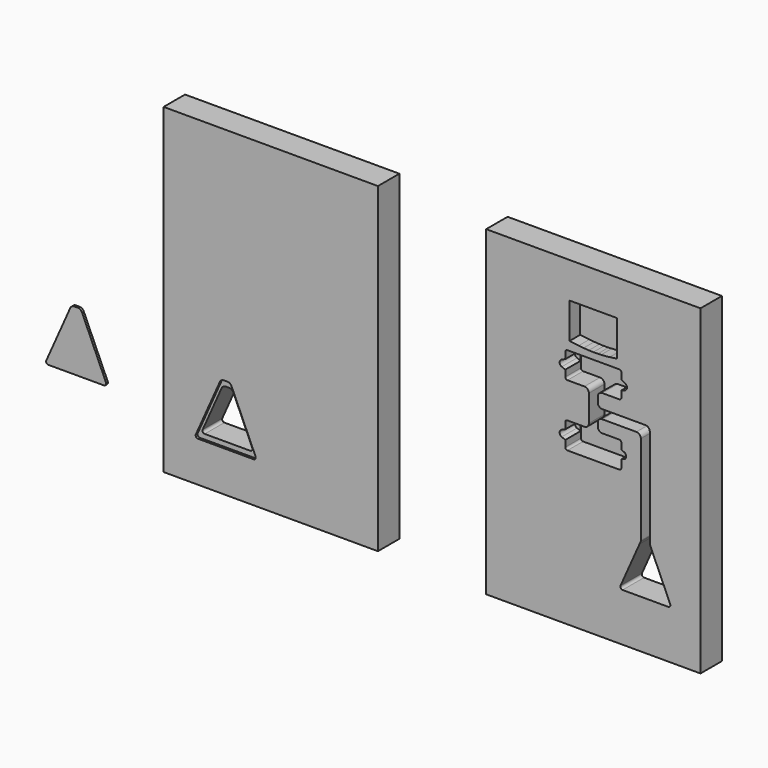
from build123d import *

# Parameters (mm, degrees)
F1_DEPTH = 38.1
F0_W     = 304.8
F0_H     = 457.2
F2_DEPTH = 10.383012
F3_DEPTH = 10.891012
F4_DEPTH = 19.05
F5_DEPTH = 34.925
F6_DEPTH = 3.175


# Not quite as in the source:
# - a feature names something its author has since deleted; it is built from what else it names


with BuildPart() as f1:
    # F0 (on Front) → F1 (new body)
    with BuildSketch(Plane.XZ):
        Polygon((-152.3615987246, 208.8922339559), (-152.3615987246, -197.5077660441), (152.4384012754, -197.5077660441), (152.4384012754, 208.8922339559), (152.4384012754, 259.6922339559), (-152.3615987246, 259.6922339559), align=None)
        with BuildLine():
            ThreePointArc((-39.8395987246, 54.7480871081), (-38.9468601937, 56.9033485772), (-36.7915987246, 57.7960871081))
            Line((-36.7915987246, 57.7960871081), (-12.6615987246, 57.7960871081))
            ThreePointArc((-12.6615987246, 57.7960871081), (-8.1714706641, 59.6559590476), (-6.3115987246, 64.1460871081))
            Line((-6.3115987246, 64.1460871081), (-6.3115987246, 101.8113421874))
            ThreePointArc((-6.3115987246, 101.8113421874), (-8.1714706641, 106.3014702479), (-12.6615987246, 108.1613421874))
            Line((-12.6615987246, 108.1613421874), (-36.7915987246, 108.1613421874))
            ThreePointArc((-36.7915987246, 108.1613421874), (-38.9468601937, 109.0540807183), (-39.8395987246, 111.2093421874))
            Line((-39.8395987246, 111.2093421874), (-39.8395987246, 120.3533421874))
            Line((-39.8395987246, 120.3533421874), (-44.9068001558, 122.3898638359))
            ThreePointArc((-44.9068001558, 122.3898638359), (-47.9325949829, 126.7961256548), (-45.0389055671, 131.2902483852))
            Line((-45.0389055671, 131.2902483852), (-39.8395987246, 133.5613421874))
            Line((-39.8395987246, 133.5613421874), (-39.8395987246, 142.7053421874))
            ThreePointArc((-39.8395987246, 142.7053421874), (-38.9468601937, 144.8606036565), (-36.7915987246, 145.7533421874))
            Line((-36.7915987246, 145.7533421874), (36.8684012754, 145.7533421874))
            ThreePointArc((36.8684012754, 145.7533421874), (39.0236627444, 144.8606036565), (39.9164012754, 142.7053421874))
            Line((39.9164012754, 142.7053421874), (39.9164012754, 133.5613421874))
            Line((39.9164012754, 133.5613421874), (45.3107705248, 130.8709577364))
            ThreePointArc((45.3107705248, 130.8709577364), (47.971895997, 126.2269453196), (44.7102550148, 121.9831100014))
            Line((44.7102550148, 121.9831100014), (39.9164012754, 120.3533421874))
            Line((39.9164012754, 120.3533421874), (39.9164012754, 111.2093421874))
            ThreePointArc((39.9164012754, 111.2093421874), (39.0236627444, 109.0540807183), (36.8684012754, 108.1613421874))
            Line((36.8684012754, 108.1613421874), (12.7384012754, 108.1613421874))
            ThreePointArc((12.7384012754, 108.1613421874), (8.2482732148, 106.3014702479), (6.3884012754, 101.8113421874))
            Line((6.3884012754, 101.8113421874), (6.3884012754, 94.3961942077))
            ThreePointArc((6.3884012754, 94.3961942077), (8.2482732148, 89.9060661471), (12.7384012754, 88.0461942077))
            Line((12.7384012754, 88.0461942077), (74.0134524345, 88.0461942077))
            ThreePointArc((74.0134524345, 88.0461942077), (78.5035804951, 86.1863222682), (80.3634524345, 81.6961942077))
            Line((80.3634524345, 81.6961942077), (80.3634524345, -58.6699053777))
            ThreePointArc((80.3634524345, -58.6699053777), (80.4325272219, -59.3285809984), (80.636746024, -59.9585965382))
            Line((80.636746024, -59.9585965382), (82.3530235747, -63.8230861254))
            Line((82.3530235747, -63.8230861254), (109.3096483672, -124.5204924261))
            ThreePointArc((109.3096483672, -124.5204924261), (109.0699167345, -127.5396503684), (106.4079419567, -128.9841835866))
            Line((106.4079419567, -128.9841835866), (41.6189629411, -128.9841835866))
            ThreePointArc((41.6189629411, -128.9841835866), (38.9569881637, -127.5396503689), (38.71725653, -124.5204924274))
            Line((38.71725653, -124.5204924274), (65.6738799598, -63.8230891221))
            Line((65.6738799598, -63.8230891221), (67.3901588456, -59.9585965238))
            ThreePointArc((67.3901588456, -59.9585965238), (67.5943776474, -59.3285809846), (67.6634524345, -58.6699053646))
            Line((67.6634524345, -58.6699053646), (67.6634524345, 68.9961942077))
            ThreePointArc((67.6634524345, 68.9961942077), (65.8035804951, 73.4863222682), (61.3134524345, 75.3461942077))
            Line((61.3134524345, 75.3461942077), (12.7384012754, 75.3461942077))
            ThreePointArc((12.7384012754, 75.3461942077), (8.2482732148, 73.4863222682), (6.3884012754, 68.9961942077))
            Line((6.3884012754, 68.9961942077), (6.3884012754, 64.1460871081))
            ThreePointArc((6.3884012754, 64.1460871081), (8.2482732148, 59.6559590476), (12.7384012754, 57.7960871081))
            Line((12.7384012754, 57.7960871081), (36.8684012754, 57.7960871081))
            ThreePointArc((36.8684012754, 57.7960871081), (39.0236627444, 56.9033485772), (39.9164012754, 54.7480871081))
            Line((39.9164012754, 54.7480871081), (39.9164012754, 46.109277755))
            Line((39.9164012754, 46.109277755), (43.96140623, 44.2832229296))
            ThreePointArc((43.96140623, 44.2832229296), (46.7916957267, 39.5734450714), (43.3787809435, 35.2671056989))
            Line((43.3787809435, 35.2671056989), (39.9164012754, 34.2150628567))
            Line((39.9164012754, 34.2150628567), (39.9164012754, 23.2520871081))
            ThreePointArc((39.9164012754, 23.2520871081), (39.0236627444, 21.0968256391), (36.8684012754, 20.2040871081))
            Line((36.8684012754, 20.2040871081), (-36.7915987246, 20.2040871081))
            ThreePointArc((-36.7915987246, 20.2040871081), (-38.9468601937, 21.0968256391), (-39.8395987246, 23.2520871081))
            Line((-39.8395987246, 23.2520871081), (-39.8395987246, 32.3960871081))
            Line((-39.8395987246, 32.3960871081), (-44.9748439025, 34.5495770214))
            ThreePointArc((-44.9748439025, 34.5495770214), (-47.9345009629, 39.0000871081), (-44.9748439025, 43.4505971948))
            Line((-44.9748439025, 43.4505971948), (-39.8395987246, 45.6040871081))
            Line((-39.8395987246, 45.6040871081), (-39.8395987246, 54.7480871081))
        make_face(mode=Mode.SUBTRACT)
        with BuildLine():
            Line((-33.9615987246, 158.0922339559), (-33.9615987246, 208.8922339559))
            Line((-33.9615987246, 208.8922339559), (34.0384012754, 208.8922339559))
            Line((34.0384012754, 208.8922339559), (34.0384012754, 158.0922339559))
            Line((34.0384012754, 158.0922339559), (23.3260869573, 156.6179031113))
            ThreePointArc((23.3260869573, 156.6179031113), (17.2149941307, 155.9271477939), (11.0776263788, 155.5330468895))
            Line((11.0776263788, 155.5330468895), (6.4386830968, 155.3478068769))
            ThreePointArc((6.4386830968, 155.3478068769), (3.2391353497, 155.2604098839), (0.0384012754, 155.2536714428))
            ThreePointArc((0.0384012754, 155.2536714428), (-3.1597948462, 155.3275354421), (-6.3551158942, 155.481930138))
            Line((-6.3551158942, 155.481930138), (-13.8442012243, 155.9384031377))
            ThreePointArc((-13.8442012243, 155.9384031377), (-17.3532100885, 156.2011225853), (-20.8535934731, 156.5609571003))
            Line((-20.8535934731, 156.5609571003), (-33.9615987246, 158.0922339559))
        make_face(mode=Mode.SUBTRACT)
    extrude(amount=F1_DEPTH)

    # F0 (on Front) → F4 (join)
    with BuildSketch(Plane.XZ):
        Polygon((34.0384012754, 208.8922339559), (-33.9615987246, 208.8922339559), (-33.9615987246, 158.0922339559), (0.0384012754, 158.0922339559), (34.0384012754, 158.0922339559), align=None)
        with BuildLine():
            Line((0.0384012754, 158.0922339559), (-33.9615987246, 158.0922339559))
            Line((-33.9615987246, 158.0922339559), (-20.8535934731, 156.5609571003))
            ThreePointArc((-20.8535934731, 156.5609571003), (-17.3532100885, 156.2011225853), (-13.8442012243, 155.9384031377))
            Line((-13.8442012243, 155.9384031377), (-6.3551158942, 155.481930138))
            ThreePointArc((-6.3551158942, 155.481930138), (-3.1597948462, 155.3275354421), (0.0384012754, 155.2536714428))
            Line((0.0384012754, 155.2536714428), (0.0384012754, 158.0922339559))
        make_face()
        with BuildLine():
            Line((34.0384012754, 158.0922339559), (0.0384012754, 158.0922339559))
            Line((0.0384012754, 158.0922339559), (0.0384012754, 155.2536714428))
            ThreePointArc((0.0384012754, 155.2536714428), (3.2391353497, 155.2604098839), (6.4386830968, 155.3478068769))
            Line((6.4386830968, 155.3478068769), (11.0776263788, 155.5330468895))
            ThreePointArc((11.0776263788, 155.5330468895), (17.2149941307, 155.9271477939), (23.3260869573, 156.6179031113))
            Line((23.3260869573, 156.6179031113), (34.0384012754, 158.0922339559))
        make_face()
    extrude(amount=F4_DEPTH)


with BuildPart() as f1b:
    # F0 (on Front) → F1, piece 2 (new body)
    with BuildSketch(Plane.XZ):
        with Locations((-458.7099272966, 34.9731193542)):
            Rectangle(F0_W, F0_H)
        with BuildLine():
            ThreePointArc((-531.1078904651, -54.6546526287), (-528.7654112075, -51.9080853942), (-525.304477644, -50.8820349497))
            Line((-525.304477644, -50.8820349497), (-520.3137643819, -50.8820349497))
            ThreePointArc((-520.3137643819, -50.8820349497), (-516.8528308173, -51.908085395), (-514.5103515598, -54.6546526313))
            Line((-514.5103515598, -54.6546526313), (-480.3611797749, -131.5472967626))
            ThreePointArc((-480.3611797749, -131.5472967626), (-480.6009114086, -134.5664547041), (-483.262886186, -136.0109879218))
            Line((-483.262886186, -136.0109879218), (-562.3553558811, -136.0109879218))
            ThreePointArc((-562.3553558811, -136.0109879218), (-565.0173306588, -134.5664547035), (-565.2570622916, -131.5472967613))
            Line((-565.2570622916, -131.5472967613), (-531.1078904651, -54.6546526287))
        make_face(mode=Mode.SUBTRACT)
    extrude(amount=F1_DEPTH)

    # F0 (on Front) → F5 (join)
    with BuildSketch(Plane.XZ):
        with BuildLine():
            Line((-520.3137643819, -50.8820349497), (-525.304477644, -50.8820349497))
            ThreePointArc((-525.304477644, -50.8820349497), (-528.7654112075, -51.9080853942), (-531.1078904651, -54.6546526287))
            Line((-531.1078904651, -54.6546526287), (-565.2570622916, -131.5472967613))
            ThreePointArc((-565.2570622916, -131.5472967613), (-565.0173306588, -134.5664547035), (-562.3553558811, -136.0109879218))
            Line((-562.3553558811, -136.0109879218), (-483.262886186, -136.0109879218))
            ThreePointArc((-483.262886186, -136.0109879218), (-480.6009114086, -134.5664547041), (-480.3611797749, -131.5472967626))
            Line((-480.3611797749, -131.5472967626), (-514.5103515598, -54.6546526313))
            ThreePointArc((-514.5103515598, -54.6546526313), (-516.8528308173, -51.908085395), (-520.3137643819, -50.8820349497))
        make_face()
        with BuildLine():
            ThreePointArc((-520.3137643868, -59.9585965283), (-516.8528308182, -60.9846469717), (-514.5103515578, -63.7312142099))
            Line((-514.5103515578, -63.7312142099), (-487.5129251071, -124.5204924274))
            ThreePointArc((-487.5129251071, -124.5204924274), (-487.7526567409, -127.5396503689), (-490.4146315182, -128.9841835866))
            Line((-490.4146315182, -128.9841835866), (-555.2036105339, -128.9841835866))
            ThreePointArc((-555.2036105339, -128.9841835866), (-557.8655853116, -127.5396503684), (-558.1053169444, -124.5204924261))
            Line((-558.1053169444, -124.5204924261), (-531.1078904631, -63.7312142127))
            ThreePointArc((-531.1078904631, -63.7312142127), (-528.7654112084, -60.9846469801), (-525.3044776489, -59.9585965337))
            Line((-525.3044776489, -59.9585965337), (-520.3137643868, -59.9585965283))
        make_face(mode=Mode.SUBTRACT)
    extrude(amount=F5_DEPTH)


with BuildPart() as f2:
    # F0 (on Front) → F2 (new body)
    with BuildSketch(Plane.XZ):
        with BuildLine():
            Line((-12.6615987246, 57.7960871081), (-36.7915987246, 57.7960871081))
            ThreePointArc((-36.7915987246, 57.7960871081), (-38.9468601937, 56.9033485772), (-39.8395987246, 54.7480871081))
            Line((-39.8395987246, 54.7480871081), (-39.8395987246, 45.6040871081))
            Line((-39.8395987246, 45.6040871081), (-39.8395987246, 32.3960871081))
            Line((-39.8395987246, 32.3960871081), (-39.8395987246, 23.2520871081))
            ThreePointArc((-39.8395987246, 23.2520871081), (-38.9468601937, 21.0968256391), (-36.7915987246, 20.2040871081))
            Line((-36.7915987246, 20.2040871081), (36.8684012754, 20.2040871081))
            ThreePointArc((36.8684012754, 20.2040871081), (39.0236627444, 21.0968256391), (39.9164012754, 23.2520871081))
            Line((39.9164012754, 23.2520871081), (39.9164012754, 34.2150628567))
            Line((39.9164012754, 34.2150628567), (39.9164012754, 46.109277755))
            Line((39.9164012754, 46.109277755), (39.9164012754, 54.7480871081))
            ThreePointArc((39.9164012754, 54.7480871081), (39.0236627444, 56.9033485772), (36.8684012754, 57.7960871081))
            Line((36.8684012754, 57.7960871081), (12.7384012754, 57.7960871081))
            ThreePointArc((12.7384012754, 57.7960871081), (8.2482732148, 59.6559590476), (6.3884012754, 64.1460871081))
            Line((6.3884012754, 64.1460871081), (6.3884012754, 68.9961942077))
            ThreePointArc((6.3884012754, 68.9961942077), (8.2482732148, 73.4863222682), (12.7384012754, 75.3461942077))
            Line((12.7384012754, 75.3461942077), (61.3134524345, 75.3461942077))
            ThreePointArc((61.3134524345, 75.3461942077), (65.8035804951, 73.4863222682), (67.6634524345, 68.9961942077))
            Line((67.6634524345, 68.9961942077), (67.6634524345, -58.6699053646))
            ThreePointArc((67.6634524345, -58.6699053646), (67.5943776474, -59.3285809846), (67.3901588456, -59.9585965238))
            Line((67.3901588456, -59.9585965238), (65.6738799598, -63.8230891221))
            ThreePointArc((65.6738799598, -63.8230891221), (68.0537799335, -61.0934782687), (71.5387284099, -60.1086770641))
            Line((71.5387284099, -60.1086770641), (76.5293692429, -60.0817894978))
            ThreePointArc((76.5293692429, -60.0817894978), (79.9957807818, -61.0891788916), (82.3530235747, -63.8230861254))
            Line((82.3530235747, -63.8230861254), (80.636746024, -59.9585965382))
            ThreePointArc((80.636746024, -59.9585965382), (80.4325272219, -59.3285809984), (80.3634524345, -58.6699053777))
            Line((80.3634524345, -58.6699053777), (80.3634524345, 81.6961942077))
            ThreePointArc((80.3634524345, 81.6961942077), (78.5035804951, 86.1863222682), (74.0134524345, 88.0461942077))
            Line((74.0134524345, 88.0461942077), (12.7384012754, 88.0461942077))
            ThreePointArc((12.7384012754, 88.0461942077), (8.2482732148, 89.9060661471), (6.3884012754, 94.3961942077))
            Line((6.3884012754, 94.3961942077), (6.3884012754, 101.8113421874))
            ThreePointArc((6.3884012754, 101.8113421874), (8.2482732148, 106.3014702479), (12.7384012754, 108.1613421874))
            Line((12.7384012754, 108.1613421874), (36.8684012754, 108.1613421874))
            ThreePointArc((36.8684012754, 108.1613421874), (39.0236627444, 109.0540807183), (39.9164012754, 111.2093421874))
            Line((39.9164012754, 111.2093421874), (39.9164012754, 120.3533421874))
            Line((39.9164012754, 120.3533421874), (39.9164012754, 133.5613421874))
            Line((39.9164012754, 133.5613421874), (39.9164012754, 142.7053421874))
            ThreePointArc((39.9164012754, 142.7053421874), (39.0236627444, 144.8606036565), (36.8684012754, 145.7533421874))
            Line((36.8684012754, 145.7533421874), (-36.7915987246, 145.7533421874))
            ThreePointArc((-36.7915987246, 145.7533421874), (-38.9468601937, 144.8606036565), (-39.8395987246, 142.7053421874))
            Line((-39.8395987246, 142.7053421874), (-39.8395987246, 133.5613421874))
            Line((-39.8395987246, 133.5613421874), (-39.8395987246, 120.3533421874))
            Line((-39.8395987246, 120.3533421874), (-39.8395987246, 111.2093421874))
            ThreePointArc((-39.8395987246, 111.2093421874), (-38.9468601937, 109.0540807183), (-36.7915987246, 108.1613421874))
            Line((-36.7915987246, 108.1613421874), (-12.6615987246, 108.1613421874))
            ThreePointArc((-12.6615987246, 108.1613421874), (-8.1714706641, 106.3014702479), (-6.3115987246, 101.8113421874))
            Line((-6.3115987246, 101.8113421874), (-6.3115987246, 64.1460871081))
            ThreePointArc((-6.3115987246, 64.1460871081), (-8.1714706641, 59.6559590476), (-12.6615987246, 57.7960871081))
        make_face()
    extrude(amount=F2_DEPTH)


with BuildPart() as f3:
    # F0 (on Front) → F3 (new body)
    with BuildSketch(Plane.XZ):
        with BuildLine():
            Line((-44.9068001558, 122.3898638359), (-39.8395987246, 120.3533421874))
            Line((-39.8395987246, 120.3533421874), (-39.8395987246, 133.5613421874))
            Line((-39.8395987246, 133.5613421874), (-45.0389055671, 131.2902483852))
            ThreePointArc((-45.0389055671, 131.2902483852), (-47.9325949829, 126.7961256548), (-44.9068001558, 122.3898638359))
        make_face()
    extrude(amount=F3_DEPTH)


with BuildPart() as f3b:
    # F0 (on Front) → F3, piece 2 (new body)
    with BuildSketch(Plane.XZ):
        with BuildLine():
            Line((45.3107705248, 130.8709577364), (39.9164012754, 133.5613421874))
            Line((39.9164012754, 133.5613421874), (39.9164012754, 120.3533421874))
            Line((39.9164012754, 120.3533421874), (44.7102550148, 121.9831100014))
            ThreePointArc((44.7102550148, 121.9831100014), (47.971895997, 126.2269453196), (45.3107705248, 130.8709577364))
        make_face()
    extrude(amount=F3_DEPTH)


with BuildPart() as f3c:
    # F0 (on Front) → F3, piece 3 (new body)
    with BuildSketch(Plane.XZ):
        with BuildLine():
            Line((-39.8395987246, 32.3960871081), (-39.8395987246, 45.6040871081))
            Line((-39.8395987246, 45.6040871081), (-44.9748439025, 43.4505971948))
            ThreePointArc((-44.9748439025, 43.4505971948), (-47.9345009629, 39.0000871081), (-44.9748439025, 34.5495770214))
            Line((-44.9748439025, 34.5495770214), (-39.8395987246, 32.3960871081))
        make_face()
    extrude(amount=F3_DEPTH)


with BuildPart() as f3d:
    # F0 (on Front) → F3, piece 4 (new body)
    with BuildSketch(Plane.XZ):
        with BuildLine():
            Line((39.9164012754, 46.109277755), (39.9164012754, 34.2150628567))
            Line((39.9164012754, 34.2150628567), (43.3787809435, 35.2671056989))
            ThreePointArc((43.3787809435, 35.2671056989), (46.7916957267, 39.5734450714), (43.96140623, 44.2832229296))
            Line((43.96140623, 44.2832229296), (39.9164012754, 46.109277755))
        make_face()
    extrude(amount=F3_DEPTH)


with BuildPart() as f6:
    # F0 (on Front) → F6 (new body)
    with BuildSketch(Plane.XZ):
        with BuildLine():
            Line((-721.0326296334, -131.5472967613), (-755.18180146, -54.6546526287))
            ThreePointArc((-755.18180146, -54.6546526287), (-757.5242807175, -51.9080853942), (-760.985214281, -50.8820349497))
            Line((-760.985214281, -50.8820349497), (-765.9759275431, -50.8820349497))
            ThreePointArc((-765.9759275431, -50.8820349497), (-769.4368611078, -51.908085395), (-771.7793403653, -54.6546526313))
            Line((-771.7793403653, -54.6546526313), (-805.9285121501, -131.5472967626))
            ThreePointArc((-805.9285121501, -131.5472967626), (-805.6887805164, -134.5664547041), (-803.0268057391, -136.0109879218))
            Line((-803.0268057391, -136.0109879218), (-723.9343360439, -136.0109879218))
            ThreePointArc((-723.9343360439, -136.0109879218), (-721.2723612662, -134.5664547035), (-721.0326296334, -131.5472967613))
        make_face()
    extrude(amount=F6_DEPTH)


solid = Compound([f1.part, f1b.part, f2.part, f3.part, f3b.part, f3c.part, f3d.part, f6.part])
